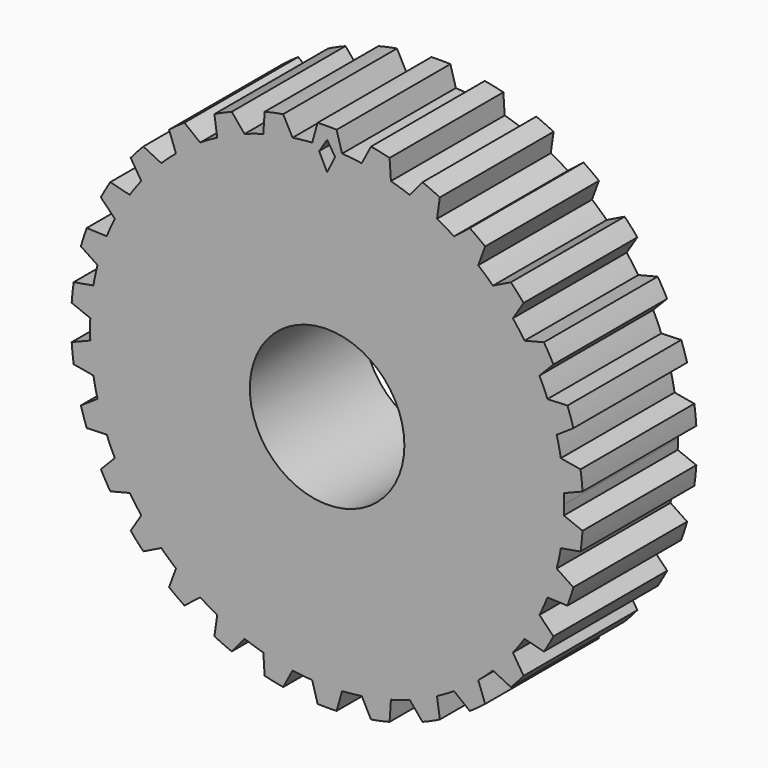
from build123d import *

# Parameters (mm, degrees)
F0_R            = 2.0701
F1_DEPTH        = 1.905
F1_COPIES_COUNT = 30
F4_DEPTH        = 12.7


# Not quite as in the source:
# - a feature of the source that left no trace in its solid (it failed there, or was rolled back) is left out
# - a pattern or mirror of a feature is missing from the dataset's text; its kind, count and spacing are read off the source's solid


with BuildPart() as f1:
    # F0 (on Front) → F1 (new body, symmetric)
    with BuildSketch(Plane.XZ):
        with BuildLine():
            ThreePointArc((-0.4003660776, 6.3373659358), (0, 6.35), (0.4003660776, 6.3373659358))
            Line((0.4003660776, 6.3373659358), (0.2543137736, 6.8532830457))
            ThreePointArc((0.2543137736, 6.8532830457), (0, 6.858), (-0.2543137736, 6.8532830457))
            Line((-0.2543137736, 6.8532830457), (-0.4003660776, 6.3373659358))
        make_face()
        with BuildLine():
            ThreePointArc((-0.4003660776, 6.3373659358), (-4.3462728519, -4.6295153414), (6.35, 0))
            ThreePointArc((6.35, 0), (4.6295153414, 4.3462728519), (0.4003660776, 6.3373659358))
            ThreePointArc((0.4003660776, 6.3373659358), (0, 6.35), (-0.4003660776, 6.3373659358))
        make_face()
        Circle(F0_R, mode=Mode.SUBTRACT)
    extrude(amount=F1_DEPTH, both=True)

    # F1_copies: F1 ×30 about axis
    f1_copies_axis = Axis((0, 0, 0), (0, 1, 0))


with BuildPart() as f1_1:
    add(f1.part)
    for i in range(1, F1_COPIES_COUNT):
        add(f1.part.rotate(f1_copies_axis, i * 360 / F1_COPIES_COUNT))

    # F3 (on Front) → F4 (cut, symmetric)
    with BuildSketch(Plane.XZ):
        Polygon((0.2138083364, 6.1984285712), (0, 6.5350458026), (0, 5.7670017704), align=None)
        Polygon((0, 5.7670017704), (0, 6.5350458026), (-0.2138083364, 6.1984285712), align=None)
    extrude(amount=F4_DEPTH, both=True, mode=Mode.SUBTRACT)


solid = f1_1.part
